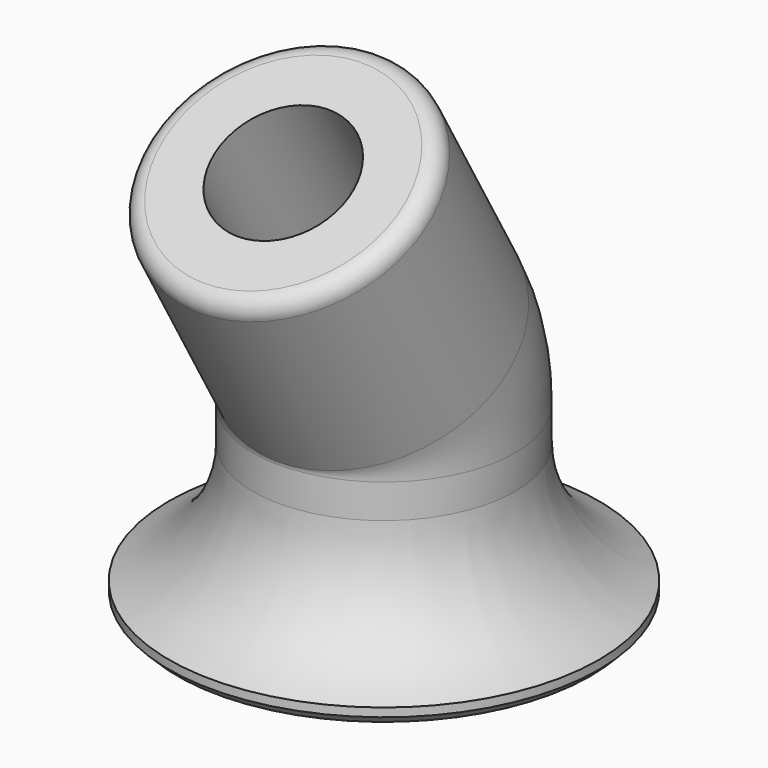
from build123d import *

# Parameters (mm, degrees)
F0_R     = 5
F0_R_2   = 3
F1_DEPTH = 0.4
F3_R     = 3.05
F3_R_2   = 1.525
F6_SIZE  = 0.2
F7_R     = 0.4


# Not quite as in the source:
# - a fillet or chamfer that OpenCascade refuses, or shapes differently, is made with other operations: its cross-section is extruded or revolved along the edge and cut away or added


with BuildPart() as f1:
    # F0 (on Top) → F1 (new body)
    with BuildSketch(Plane.XY):
        Circle(F0_R)
        Circle(F0_R_2, mode=Mode.SUBTRACT)
    extrude(amount=F1_DEPTH)

    # F4: sweep along a path in F2
    with BuildLine(Plane.YZ) as f4_path:
        Line((0, 0), (0, 4))
        ThreePointArc((0, 4), (-0.1090373559, 4.8282209443), (-0.4287187079, 5.6))
        Line((-0.4287187079, 5.6), (-2.9287187079, 9.9301270189))
    # F3 (on Top) → F4 (sweep)
    with BuildSketch(Plane.XY):
        Circle(F3_R)
        Circle(F3_R_2, mode=Mode.SUBTRACT)
    sweep(path=f4_path.line)

    # F5: fillet of radius 3 on 1 edges, made by hand

    # F5_s1 → F5_t2 (revolve)
    with BuildSketch(Plane.XZ):
        with BuildLine():
            ThreePointArc((5, 0.4), (3.5852484912, 1.4999859616), (3.05, 3.2102490993))
            Line((3.05, 3.2102490993), (3.05, 0.4))
            Line((3.05, 0.4), (5, 0.4))
        make_face()
    revolve(axis=Axis((0, 0, 0.4), (0, 0, 1)))

    # F6
    f6_edges = [f1.edges().sort_by_distance(p)[0] for p in [
        (-5, 0, 0),
        (-1.525, 0, 0),
    ]]
    chamfer(f6_edges, length=F6_SIZE)

    # F7
    f7_edges = [f1.edges().sort_by_distance(p)[0] for p in [
        (-3.05, -2.928719, 9.930127),
    ]]
    fillet(f7_edges, radius=F7_R)


solid = f1.part
